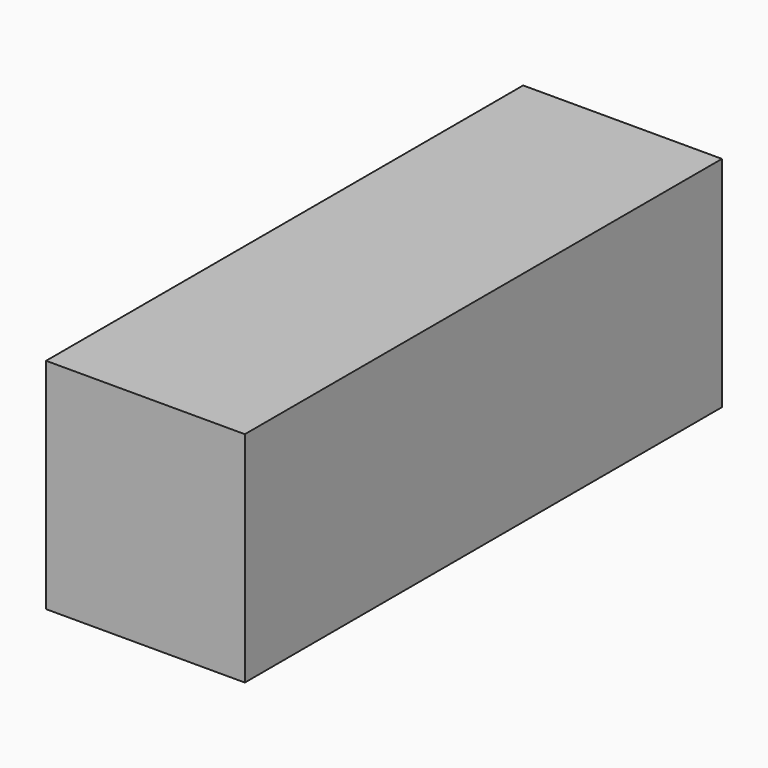
from build123d import *

# Parameters (mm, degrees)
F0_W          = 150
F0_H          = 55
F1_DEPTH      = 25
F1_DEPTH_BACK = 25


# Not quite as in the source:
# - a feature of the source that left no trace in its solid (it failed there, or was rolled back) is left out


with BuildPart() as f1:
    # F0 (on Right) → F1 (new body, two sides)
    with BuildSketch(Plane.YZ) as f1_sk:
        Rectangle(F0_W, F0_H)
    extrude(amount=F1_DEPTH)
    extrude(f1_sk.sketch, amount=-F1_DEPTH_BACK)


solid = f1.part
